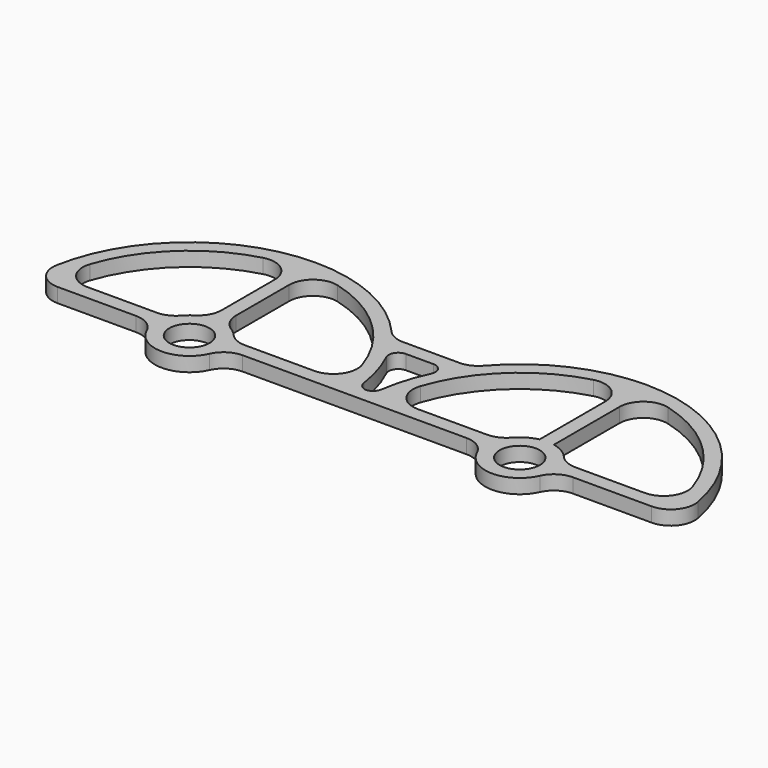
from build123d import *

# Parameters (mm, degrees)
F0_R        = 4.2
F1_DEPTH    = 3
F3_DEPTH    = 3
F4_R        = 5
F5_T1_DEPTH = 3


# Not quite as in the source:
# - a fillet or chamfer that OpenCascade refuses, or shapes differently, is made with other operations: its cross-section is extruded or revolved along the edge and cut away or added


with BuildPart() as f1:
    # F0 (on Top) → F1 (new body)
    with BuildSketch(Plane.XY):
        with BuildLine():
            ThreePointArc((6.5452272688, 3), (7.0344024741, 1.5353116402), (7.2, 0))
            Line((7.2, 0), (33, 0))
            Line((33, 0), (36, 0))
            Line((36, 0), (61.8, 0))
            ThreePointArc((61.8, 0), (61.9655975259, 1.5353116402), (62.4547727312, 3))
            Line((62.4547727312, 3), (39.1503768868, 3))
            ThreePointArc((39.1503768868, 3), (69, 30), (98.8496231132, 3))
            Line((98.8496231132, 3), (75.5452272688, 3))
            ThreePointArc((75.5452272688, 3), (76.0344024741, 1.5353116402), (76.2, 0))
            Line((76.2, 0), (102, 0))
            ThreePointArc((102, 0), (79.5543660777, 31.2666812549), (42.7511905032, 20))
            Line((42.7511905032, 20), (26.2488094968, 20))
            ThreePointArc((26.2488094968, 20), (-10.5543660777, 31.2666812549), (-33, 0))
            Line((-33, 0), (-7.2, 0))
            ThreePointArc((-7.2, 0), (-7.0344024741, 1.5353116402), (-6.5452272688, 3))
            Line((-6.5452272688, 3), (-29.8496231132, 3))
            ThreePointArc((-29.8496231132, 3), (0, 30), (29.8496231132, 3))
            Line((29.8496231132, 3), (6.5452272688, 3))
        make_face()
        with BuildLine():
            Line((36.1366465497, 3), (32.8633534503, 3))
            ThreePointArc((32.8633534503, 3), (31.364916731, 10.2587522855), (28.2842712475, 17))
            Line((28.2842712475, 17), (40.7157287525, 17))
            ThreePointArc((40.7157287525, 17), (37.635083269, 10.2587522855), (36.1366465497, 3))
        make_face(mode=Mode.SUBTRACT)
        with BuildLine():
            ThreePointArc((-7.2, 0), (0, -7.2), (7.2, 0))
            ThreePointArc((7.2, 0), (7.0344024741, 1.5353116402), (6.5452272688, 3))
            ThreePointArc((6.5452272688, 3), (0, 7.2), (-6.5452272688, 3))
            ThreePointArc((-6.5452272688, 3), (-7.0344024741, 1.5353116402), (-7.2, 0))
        make_face()
        Circle(F0_R, mode=Mode.SUBTRACT)
        with BuildLine():
            ThreePointArc((62.4547727312, 3), (61.9655975259, 1.5353116402), (61.8, 0))
            ThreePointArc((61.8, 0), (69, -7.2), (76.2, 0))
            ThreePointArc((76.2, 0), (76.0344024741, 1.5353116402), (75.5452272688, 3))
            ThreePointArc((75.5452272688, 3), (69, 7.2), (62.4547727312, 3))
        make_face()
        with Locations((69, 0)):
            Circle(F0_R, mode=Mode.SUBTRACT)
    extrude(amount=F1_DEPTH)

    # F2 (on face) → F3 (join, through all)
    with BuildSketch(Plane.XY.offset(3)):
        with BuildLine():
            Line((1.5, 7.0420167566), (1.5, 29.9624765332))
            ThreePointArc((1.5, 29.9624765332), (0.7502346317, 29.9906176662), (0, 30))
            Line((0, 30), (0, 7.2))
            ThreePointArc((0, 7.2), (0.7541483119, 7.1603952631), (1.5, 7.0420167566))
        make_face()
        with BuildLine():
            Line((0, 7.2), (0, 30))
            ThreePointArc((0, 30), (-0.7502346317, 29.9906176662), (-1.5, 29.9624765332))
            Line((-1.5, 29.9624765332), (-1.5, 7.0420167566))
            ThreePointArc((-1.5, 7.0420167566), (-0.7541483119, 7.1603952631), (0, 7.2))
        make_face()
        with BuildLine():
            Line((69, 7.2), (69, 30))
            ThreePointArc((69, 30), (68.2497653683, 29.9906176662), (67.5, 29.9624765332))
            Line((67.5, 29.9624765332), (67.5, 7.0420167566))
            ThreePointArc((67.5, 7.0420167566), (68.2458516881, 7.1603952631), (69, 7.2))
        make_face()
        with BuildLine():
            Line((70.5, 7.0420167566), (70.5, 29.9624765332))
            ThreePointArc((70.5, 29.9624765332), (69.7502346317, 29.9906176662), (69, 30))
            Line((69, 30), (69, 7.2))
            ThreePointArc((69, 7.2), (69.7541483119, 7.1603952631), (70.5, 7.0420167566))
        make_face()
    extrude(amount=-F3_DEPTH)

    # F4
    f4_edges = [f1.edges().sort_by_distance(p)[0] for p in [
        (-29.849623, 3, 1.5),
        (29.849623, 3, 1.5),
        (98.849623, 3, 1.5),
        (39.150377, 3, 1.5),
        (-7.2, 0, 1.5),
        (7.2, 0, 1.5),
        (61.8, 0, 1.5),
        (76.2, 0, 1.5),
        (75.545227, 3, 1.5),
        (62.454773, 3, 1.5),
        (-6.545227, 3, 1.5),
        (6.545227, 3, 1.5),
        (26.248809, 20, 1.5),
        (42.751191, 20, 1.5),
        (102, 0, 1.5),
        (-33, 0, 1.5),
        (-1.5, 7.042017, 1.5),
        (1.5, 7.042017, 1.5),
        (1.5, 29.962477, 1.5),
        (-1.5, 29.962477, 1.5),
        (70.5, 29.962477, 1.5),
        (67.5, 29.962477, 1.5),
    ]]
    fillet(f4_edges, radius=F4_R)

    # F5: fillet of radius 2 on 4 edges, made by hand

    # F5_s2 → F5_t1 (join)
    with BuildSketch(Plane.XY):
        with BuildLine():
            ThreePointArc((31.6227766017, 17), (29.9324680922, 16.0690449676), (29.8157607959, 14.1428571429))
            ThreePointArc((29.8157607959, 14.1428571429), (29.0851207181, 15.5902454379), (28.2842712475, 17))
            Line((28.2842712475, 17), (31.6227766017, 17))
        make_face()
        with BuildLine():
            ThreePointArc((37.3772233983, 17), (39.0675319078, 16.0690449676), (39.1842392041, 14.1428571429))
            ThreePointArc((39.1842392041, 14.1428571429), (39.9148792819, 15.5902454379), (40.7157287525, 17))
            Line((40.7157287525, 17), (37.3772233983, 17))
        make_face()
        with BuildLine():
            ThreePointArc((34.6410161514, 3), (33.33170881, 3.488142108), (32.6615295142, 4.7142857143))
            ThreePointArc((32.6615295142, 4.7142857143), (32.7736520051, 3.8584626791), (32.8633534503, 3))
            Line((32.8633534503, 3), (34.6410161514, 3))
        make_face()
        with BuildLine():
            ThreePointArc((36.3384704858, 4.7142857143), (35.66829119, 3.488142108), (34.3589838486, 3))
            Line((34.3589838486, 3), (36.1366465497, 3))
            ThreePointArc((36.1366465497, 3), (36.2263479949, 3.8584626791), (36.3384704858, 4.7142857143))
        make_face()
    extrude(amount=F5_T1_DEPTH)


solid = f1.part
